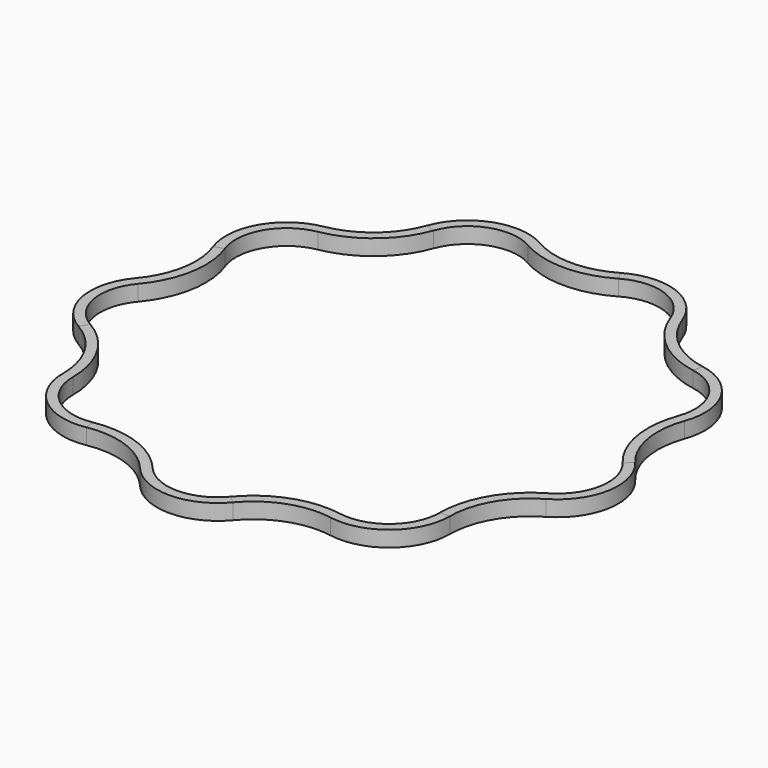
from build123d import *

# Parameters (mm, degrees)
F1_DEPTH = 16
F2_COUNT = 9
F2_ANGLE = 320


with BuildPart() as f1:
    # F0 (on Top) → F1 (new body)
    with BuildSketch(Plane.XY):
        with BuildLine():
            ThreePointArc((-1274.3186272061, 728.5859559918), (-1240.4482893018, 762.4562938962), (-1192.7306716228, 758.2815432988))
            ThreePointArc((-1192.7306716228, 758.2815432988), (-1149.3186272061, 746.6493210555), (-1105.9065827894, 758.2815432988))
            Line((-1105.9065827894, 758.2815432988), (-1108.4065827894, 762.6116703177))
            ThreePointArc((-1108.4065827894, 762.6116703177), (-1149.3186272061, 751.6493210555), (-1190.2306716228, 762.6116703177))
            ThreePointArc((-1190.2306716228, 762.6116703177), (-1242.1583900184, 767.154757), (-1279.01709031, 730.2960567085))
            Line((-1279.01709031, 730.2960567085), (-1274.3186272061, 728.5859559918))
        make_face()
        with BuildLine():
            ThreePointArc((-1105.9065827894, 758.2815432988), (-1149.3186272061, 746.6493210555), (-1192.7306716228, 758.2815432988))
            ThreePointArc((-1192.7306716228, 758.2815432988), (-1240.4482893018, 762.4562938962), (-1274.3186272061, 728.5859559918))
            Line((-1274.3186272061, 728.5859559918), (-1269.6201641022, 726.8758552752))
            ThreePointArc((-1269.6201641022, 726.8758552752), (-1238.7381885852, 757.7578307922), (-1195.2306716228, 753.9514162799))
            ThreePointArc((-1195.2306716228, 753.9514162799), (-1149.3186272061, 741.6493210555), (-1103.4065827894, 753.9514162799))
            Line((-1103.4065827894, 753.9514162799), (-1105.9065827894, 758.2815432988))
        make_face()
    extrude(amount=F1_DEPTH)


with BuildPart() as f2_1:
    # F2: instance of F1
    add(f1.part.rotate(Axis((-1149.3186272061, 512.0796050457, 0), (0, 0, 1)), 1 * F2_ANGLE / (F2_COUNT - 1)))


with BuildPart() as f2_2:
    # F2: instance of F1
    add(f1.part.rotate(Axis((-1149.3186272061, 512.0796050457, 0), (0, 0, 1)), 2 * F2_ANGLE / (F2_COUNT - 1)))


with BuildPart() as f2_3:
    # F2: instance of F1
    add(f1.part.rotate(Axis((-1149.3186272061, 512.0796050457, 0), (0, 0, 1)), 3 * F2_ANGLE / (F2_COUNT - 1)))


with BuildPart() as f2_4:
    # F2: instance of F1
    add(f1.part.rotate(Axis((-1149.3186272061, 512.0796050457, 0), (0, 0, 1)), 4 * F2_ANGLE / (F2_COUNT - 1)))


with BuildPart() as f2_5:
    # F2: instance of F1
    add(f1.part.rotate(Axis((-1149.3186272061, 512.0796050457, 0), (0, 0, 1)), 5 * F2_ANGLE / (F2_COUNT - 1)))


with BuildPart() as f2_6:
    # F2: instance of F1
    add(f1.part.rotate(Axis((-1149.3186272061, 512.0796050457, 0), (0, 0, 1)), 6 * F2_ANGLE / (F2_COUNT - 1)))


with BuildPart() as f2_7:
    # F2: instance of F1
    add(f1.part.rotate(Axis((-1149.3186272061, 512.0796050457, 0), (0, 0, 1)), 7 * F2_ANGLE / (F2_COUNT - 1)))


with BuildPart() as f2_8:
    # F2: instance of F1
    add(f1.part.rotate(Axis((-1149.3186272061, 512.0796050457, 0), (0, 0, 1)), 8 * F2_ANGLE / (F2_COUNT - 1)))


solid = Compound([f1.part, f2_1.part, f2_2.part, f2_3.part, f2_4.part, f2_5.part, f2_6.part, f2_7.part, f2_8.part])
